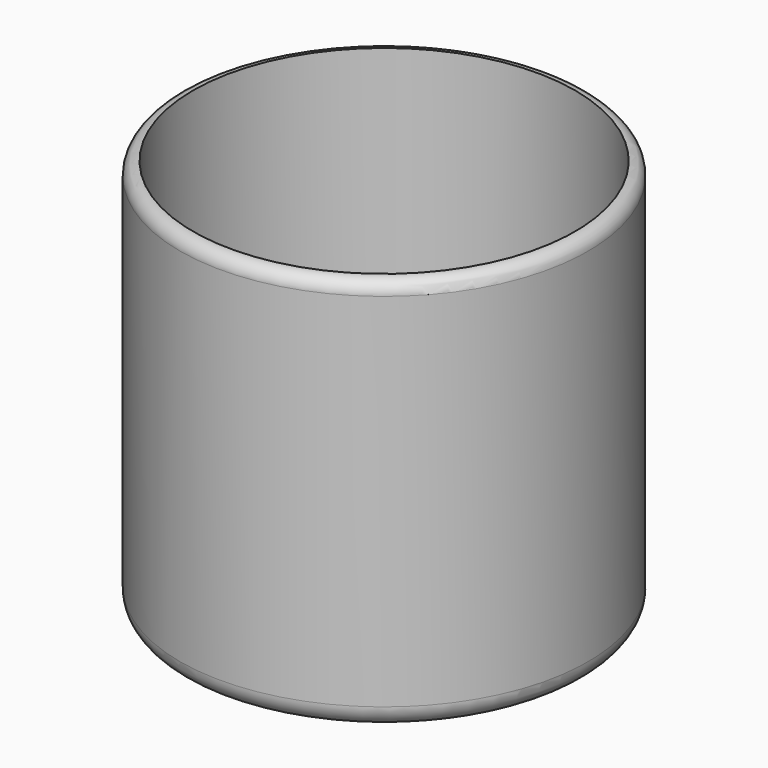
from build123d import *

# Parameters (mm, degrees)
F2_R = 2.99999
F3_R = 5


# Not quite as in the source:
# - a fillet or chamfer is up to 0.001 mm smaller than in the source, because OpenCascade refuses the exact size


with BuildPart() as f1:
    # F0 (on Front) → F1 (revolve)
    with BuildSketch(Plane.XZ):
        Polygon((-91.4914906025, 49.9999961555), (-94.4914906025, 49.9999961555), (-94.4914906025, -41.0000038445), (-47.6173348725, -41.0000038445), (-47.6173348725, -35.0000038445), (-91.4914906025, -35.0000038445), align=None)
    revolve(axis=Axis((-47.6173348725, 0, -38.0000038445), (0, 0, 1)))

    # F2 (radius 3 in the source; OpenCascade refuses exactly that, so slightly less here)
    f2_edges = [f1.edges().sort_by_distance(p)[0] for p in [
        (-0.743179, 0, 49.999996),
    ]]
    fillet(f2_edges, radius=F2_R)

    # F3
    f3_edges = [f1.edges().sort_by_distance(p)[0] for p in [
        (-0.743179, 0, -41.000004),
    ]]
    fillet(f3_edges, radius=F3_R)


solid = f1.part
